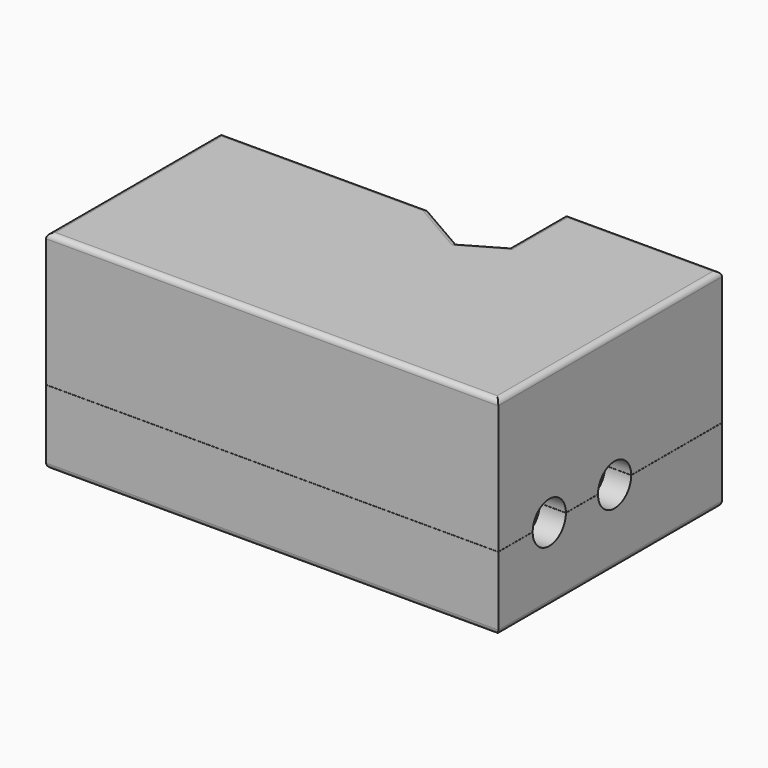
from build123d import *

# Parameters (mm, degrees)
F1_DEPTH  = 200
F2_T      = -25
F3_R      = 20
F4_DEPTH  = 25
F5_R      = 5
F6_R      = 12.5
F7_DEPTH  = 25
F8_W      = 515.9801917831
F8_H      = 0.1
F9_DEPTH  = 500
F11_DEPTH = 25
F12_R     = 50
F14_DEPTH = 30
F15_DEPTH = 0.1


with BuildPart() as f1:
    # F0 (on Top) → F1 (new body)
    with BuildSketch(Plane.XY):
        Polygon((-217.7152904997, -95), (217.7152904997, -95), (217.7152904997, 95), (217.7152904997, 174.1873925667), (67.7152904997, 174.1873925667), (67.7152904997, 105.9900790749), (33.0742743483, 85.9900790749), (-17.7152904997, 115.3134480119), (-217.7152904997, 115.3134480119), (-217.7152904997, 95), align=None)
    extrude(amount=F1_DEPTH)

    # F2
    f2_openings = [f1.faces().sort_by_distance(p)[0] for p in [
        (12.289401, 20.806229, 200),
    ]]
    offset(amount=F2_T, openings=f2_openings, kind=Kind.INTERSECTION)

    # F3 (on face) → F4 (cut)
    with BuildSketch(Plane.YZ.offset(217.7152904997)):
        with Locations((45, 71.226)):
            Circle(F3_R)
        with Locations((-33.618, 71.226)):
            Circle(F3_R)
    extrude(amount=-F4_DEPTH, mode=Mode.SUBTRACT)

    # F5
    f5_edges = [f1.edges().sort_by_distance(p)[0] for p in [
        (0, -70, 25),
        (0, -95, 200),
        (217.71529, 39.593696, 200),
        (142.71529, 174.187393, 200),
        (67.71529, 140.088736, 200),
        (50.394782, 95.990079, 200),
        (7.679492, 100.651764, 200),
        (-117.71529, 115.313448, 200),
        (-217.71529, 10.156724, 200),
        (0, -95, 0),
        (217.71529, 39.593696, 0),
        (142.71529, 174.187393, 0),
        (67.71529, 140.088736, 0),
        (50.394782, 95.990079, 0),
        (7.679492, 100.651764, 0),
        (-117.71529, 115.313448, 0),
        (-217.71529, 10.156724, 0),
        (-192.71529, -70, 112.5),
        (192.71529, -70, 112.5),
    ]]
    fillet(f5_edges, radius=F5_R)

    # F6 (on face) → F7 (cut)
    with BuildSketch(Plane(origin=(-217.7152904997, 0, 0), x_dir=(0, -1, 0), z_dir=(-1, 0, 0))):
        with Locations((-45, 71.226)):
            Circle(F6_R)
        with Locations((33.618, 71.226)):
            Circle(F6_R)
    extrude(amount=-F7_DEPTH, mode=Mode.SUBTRACT)

    # F8 (on face) → F9 (cut)
    with BuildSketch(Plane.XZ.offset(95)):
        with Locations((13.46298667, 71.23)):
            Rectangle(F8_W, F8_H)
    extrude(amount=-F9_DEPTH, mode=Mode.SUBTRACT)

    # F10 (on face) → F11 (join)
    with BuildSketch(Plane.XY.offset(200)):
        Polygon((-197.7152904997, 95.3134480119), (-212.7152904997, -90), (197.7152904997, -75), (197.7152904997, 154.1873925667), (87.7152904997, 154.1873925667), (87.7152904997, 94.4430736911), (33.0742743483, 62.8960683073), (-23.0742743483, 95.3134480119), align=None)
    extrude(amount=-F11_DEPTH)

    # F12
    f12_edges = [f1.edges().sort_by_distance(p)[0] for p in [
        (33.074274, 57.122566, 48.09),
        (33.074274, 57.122566, 123.14),
    ]]
    fillet(f12_edges, radius=F12_R)

    # F13 (on face) → F14 (cut)
    with BuildSketch(Plane(origin=(-217.7152904997, 0, 0), x_dir=(0, -1, 0), z_dir=(-1, 0, 0))):
        with BuildLine():
            Line((33.6188076483, 103.7538542444), (-44.9991923032, 103.7558062851))
            ThreePointArc((-44.9991923032, 103.7558062851), (-77.5293160692, 71.4045879899), (-45.3563629488, 38.6981457356))
            Line((-45.3563629488, 38.6981457356), (33.618, 38.6981457356))
            ThreePointArc((33.618, 38.6981457356), (66.1458542619, 71.2255961758), (33.6188076483, 103.7538542544))
        make_face()
        with BuildLine():
            ThreePointArc((-45.3558147624, 38.7981457356), (-77.4293160726, 71.4043126593), (-44.9991947862, 103.6558062851))
            Line((-44.9991947862, 103.6558062851), (33.618, 103.6538542644))
            ThreePointArc((33.618, 103.6538542644), (66.0458542644, 71.226), (33.618, 38.7981457356))
            Line((33.618, 38.7981457356), (-45.3558147624, 38.7981457356))
        make_face(mode=Mode.SUBTRACT)
    extrude(amount=-F14_DEPTH, mode=Mode.SUBTRACT)

    # F15 (add): faces of the model
    f15_faces = [f1.faces().sort_by_distance(p)[0] for p in [
        (-205.2152904997, 5.691, 71.18),
        (-205.2152904997, 67.4648445152, 71.18),
        (-205.2143249793, -56.0826160003, 71.18),
    ]]
    extrude(f15_faces, amount=F15_DEPTH)


solid = f1.part
